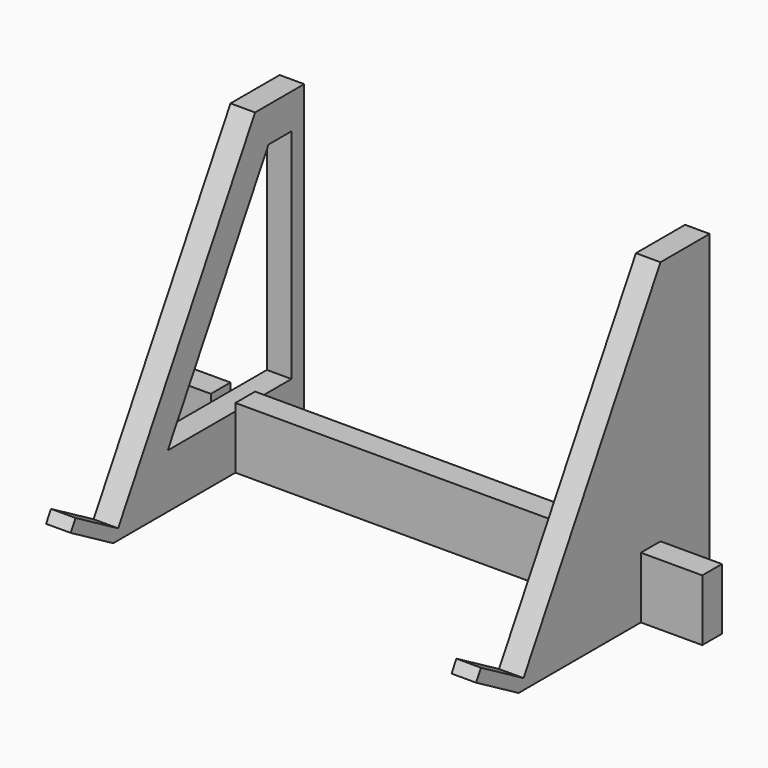
from build123d import *

# Parameters (mm, degrees)
F0_W          = 10
F0_H          = 4
F1_DEPTH      = 10
F0_W_2        = 62
F0_W_3        = 4
F0_H_2        = 10
F0_H_3        = 46
F2_DEPTH      = 50
F3_T1_DEPTH   = 452.0963970585
F3_2_T1_DEPTH = 452.0963970585
F4_W          = 4
F4_H          = 2
F5_DEPTH      = 10
F6_W          = 4
F6_H          = 2
F7_DEPTH      = 10
F8_DEPTH      = 5
F9_DEPTH      = 5
F11_DEPTH     = 25


# Not quite as in the source:
# - a fillet or chamfer that OpenCascade refuses, or shapes differently, is made with other operations: its cross-section is extruded or revolved along the edge and cut away or added


with BuildPart() as f1:
    # F0 (on Top) → F1 (new body)
    with BuildSketch(Plane.XY):
        with Locations((5, -2)):
            Rectangle(F0_W, F0_H)
    extrude(amount=F1_DEPTH)


with BuildPart() as f1b:
    # F0 (on Top) → F1, piece 2 (new body)
    with BuildSketch(Plane.XY):
        with Locations((45, -2)):
            Rectangle(F0_W_2, F0_H)
    extrude(amount=F1_DEPTH)


with BuildPart() as f1c:
    # F0 (on Top) → F1, piece 3 (new body)
    with BuildSketch(Plane.XY):
        with Locations((85, -2)):
            Rectangle(F0_W, F0_H)
    extrude(amount=F1_DEPTH)


with BuildPart() as f2:
    # F0 (on Top) → F2 (new body)
    with BuildSketch(Plane.XY):
        with Locations((12, 5)):
            Rectangle(F0_W_3, F0_H_2)
        with Locations((12, -2)):
            Rectangle(F0_W_3, F0_H)
        with Locations((12, -27)):
            Rectangle(F0_W_3, F0_H_3)
    extrude(amount=F2_DEPTH)

    # F3: chamfer of 50 x 86.6025403784 on 1 edges, made by hand

    # F3_s2 → F3_t1 (cut)
    with BuildSketch(Plane.YZ.offset(-214.0481985292)):
        Polygon((-50, -36.6025403784), (0, 50), (-50, 50), align=None)
    extrude(amount=F3_T1_DEPTH, mode=Mode.SUBTRACT)

    # F4 (on face) → F5 (join)
    with BuildSketch(Plane(origin=(0, -21.6506350946, 12.5), x_dir=(1, 0, 0), z_dir=(0, -0.8660254038, 0.5))):
        with Locations((12, -13.4337567297)):
            Rectangle(F4_W, F4_H)
    extrude(amount=F5_DEPTH)

    # F0 (on Top) → F9 (cut)
    with BuildSketch(Plane.XY):
        with Locations((12, -2)):
            Rectangle(F0_W_3, F0_H)
    extrude(amount=F9_DEPTH, mode=Mode.SUBTRACT)

    # F10 (on face) → F11 (cut)
    with BuildSketch(Plane(origin=(10, 0, 0), x_dir=(0, -1, 0), z_dir=(-1, 0, 0))):
        Polygon((-7.4024386704, 44.2947206634), (-7.4024386704, 8.7926825508), (17.7682936192, 8.7926825508), (-2.7288176419, 44.2947206634), align=None)
    extrude(amount=-F11_DEPTH, mode=Mode.SUBTRACT)


with BuildPart() as f2b:
    # F0 (on Top) → F2, piece 2 (new body)
    with BuildSketch(Plane.XY):
        with Locations((78, 5)):
            Rectangle(F0_W_3, F0_H_2)
        with Locations((78, -2)):
            Rectangle(F0_W_3, F0_H)
        with Locations((78, -27)):
            Rectangle(F0_W_3, F0_H_3)
    extrude(amount=F2_DEPTH)

    # F3#2: chamfer of 50 x 86.6025403784 on 1 edges, made by hand

    # F3_2_s2 → F3_2_t1 (cut)
    with BuildSketch(Plane.YZ.offset(-148.0481985292)):
        Polygon((-50, -36.6025403784), (0, 50), (-50, 50), align=None)
    extrude(amount=F3_2_T1_DEPTH, mode=Mode.SUBTRACT)

    # F6 (on face) → F7 (join)
    with BuildSketch(Plane(origin=(0, -21.6506350946, 12.5), x_dir=(1, 0, 0), z_dir=(0, -0.8660254038, 0.5))):
        with Locations((78, -13.4337567297)):
            Rectangle(F6_W, F6_H)
    extrude(amount=F7_DEPTH)


with BuildPart() as f8:
    # F0 (on Top) → F8 (new body)
    with BuildSketch(Plane.XY):
        with Locations((12, -2)):
            Rectangle(F0_W_3, F0_H)
    extrude(amount=F8_DEPTH)


with BuildPart() as f8b:
    # F0 (on Top) → F8, piece 2 (new body)
    with BuildSketch(Plane.XY):
        with Locations((78, -2)):
            Rectangle(F0_W_3, F0_H)
    extrude(amount=F8_DEPTH)


solid = Compound([f1.part, f1b.part, f1c.part, f2.part, f2b.part, f8.part, f8b.part])
